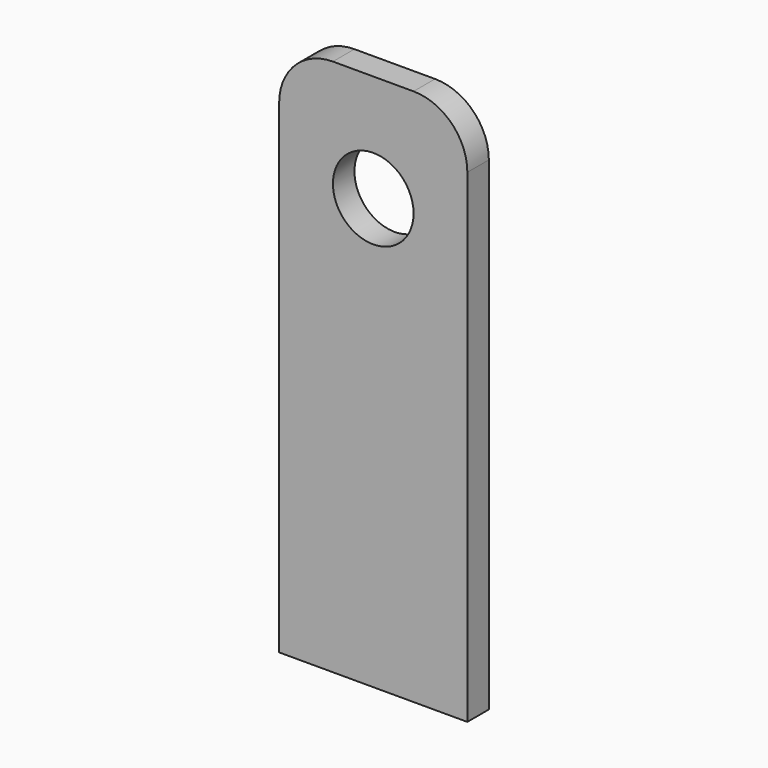
from build123d import *

# Parameters (mm, degrees)
F0_W          = 70
F0_H          = 200
F1_DEPTH      = 10
F2_R          = 15
F3_DEPTH      = 218
F3_DEPTH_BACK = 25
F4_R          = 20


# Not quite as in the source:
# - an extrude ends at something that could not be found from the text; its depth is read off the source's solid


with BuildPart() as f1:
    # F0 (on Front) → F1 (new body)
    with BuildSketch(Plane.XZ):
        Rectangle(F0_W, F0_H)
    extrude(amount=F1_DEPTH)

    # F2 (on Front) → F3 (cut, two sides)
    with BuildSketch(Plane.XZ) as f3_sk:
        with Locations((0, 60)):
            Circle(F2_R)
    extrude(amount=-F3_DEPTH, mode=Mode.SUBTRACT)
    extrude(f3_sk.sketch, amount=F3_DEPTH_BACK, mode=Mode.SUBTRACT)

    # F4
    f4_edges = [f1.edges().sort_by_distance(p)[0] for p in [
        (-35, -5, 100),
        (35, -5, 100),
    ]]
    fillet(f4_edges, radius=F4_R)


solid = f1.part
